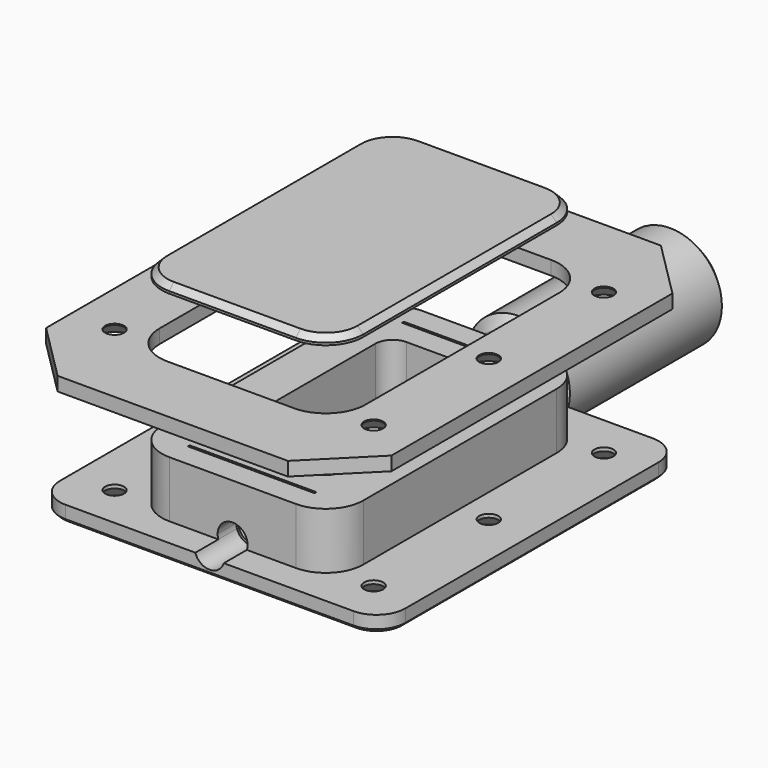
from build123d import *

# Parameters (mm, degrees)
F1_R          = 1.65
F2_DEPTH      = 2.8
F4_DEPTH      = 9.8
F6_DEPTH      = 65
F7_W          = 60
F7_H          = 81
F7_R          = 1.65
F8_DEPTH      = 2.4
F9_SIZE       = 10
F10_SIZE      = 2.2
F10_2_SIZE    = 2.2
F12_R         = 9
F12_R_2       = 2.7
F13_DEPTH     = 37
F14_SIZE      = 2
F16_SIZE      = 0.6
F19_DEPTH     = 1.4
F21_DEPTH     = 1.6
F22_W         = 11
F22_H         = 37.4000005722
F22_H_2       = 1.5999997139
F23_DEPTH     = 2
F24_SIZE      = 1.99999
F25_T1_DEPTH  = 38.2094607039
F25_T3_DEPTH  = 32
F25_T6_ANGLE  = 101.1642209188
F25_T8_ANGLE  = 101.1642209188
F25_T10_ANGLE = 101.1642209188
F25_T12_ANGLE = 101.1642209188
F26_SIZE      = 1
F27_W         = 22
F27_H         = 0.4
F28_DEPTH     = 12


# Not quite as in the source:
# - a fillet or chamfer that OpenCascade refuses, or shapes differently, is made with other operations: its cross-section is extruded or revolved along the edge and cut away or added
# - a fillet or chamfer is up to 0.001 mm smaller than in the source, because OpenCascade refuses the exact size


with BuildPart() as f2:
    # F1 (on Top) → F2 (new body)
    with BuildSketch(Plane.XY):
        with BuildLine():
            Line((25, 32.5), (-25, 32.5))
            ThreePointArc((-25, 32.5), (-28.5355339059, 31.0355339059), (-30, 27.5))
            Line((-30, 27.5), (-30, -27.5))
            ThreePointArc((-30, -27.5), (-28.5355339059, -31.0355339059), (-25, -32.5))
            Line((-25, -32.5), (25, -32.5))
            ThreePointArc((25, -32.5), (28.5355339059, -31.0355339059), (30, -27.5))
            Line((30, -27.5), (30, 27.5))
            ThreePointArc((30, 27.5), (28.5355339059, 31.0355339059), (25, 32.5))
        make_face()
        with Locations((-22.5, -25)):
            Circle(F1_R, mode=Mode.SUBTRACT)
        with Locations((22.5, -25)):
            Circle(F1_R, mode=Mode.SUBTRACT)
        with Locations((-22.5, 0)):
            Circle(F1_R, mode=Mode.SUBTRACT)
        with Locations((-22.5, 25)):
            Circle(F1_R, mode=Mode.SUBTRACT)
        with BuildLine():
            ThreePointArc((-10, 16), (-9.1213203436, 18.1213203436), (-7, 19))
            Line((-7, 19), (7, 19))
            ThreePointArc((7, 19), (9.1213203436, 18.1213203436), (10, 16))
            Line((10, 16), (10, -16))
            ThreePointArc((10, -16), (9.1213203436, -18.1213203436), (7, -19))
            Line((7, -19), (-7, -19))
            ThreePointArc((-7, -19), (-9.1213203436, -18.1213203436), (-10, -16))
            Line((-10, -16), (-10, 16))
        make_face(mode=Mode.SUBTRACT)
        with Locations((22.5, 0)):
            Circle(F1_R, mode=Mode.SUBTRACT)
        with Locations((22.5, 25)):
            Circle(F1_R, mode=Mode.SUBTRACT)
    extrude(amount=F2_DEPTH)

    # F3 (on face) → F4 (join)
    with BuildSketch(Plane.XY.offset(2.8)):
        with BuildLine():
            Line((11, 27.5), (-11, 27.5))
            ThreePointArc((-11, 27.5), (-15.5961940777, 25.5961940777), (-17.5, 21))
            Line((-17.5, 21), (-17.5, -21))
            ThreePointArc((-17.5, -21), (-15.5961940777, -25.5961940777), (-11, -27.5))
            Line((-11, -27.5), (11, -27.5))
            ThreePointArc((11, -27.5), (15.5961940777, -25.5961940777), (17.5, -21))
            Line((17.5, -21), (17.5, 21))
            ThreePointArc((17.5, 21), (15.5961940777, 25.5961940777), (11, 27.5))
        make_face()
        with BuildLine():
            Line((-10, -16), (-10, 16))
            ThreePointArc((-10, 16), (-9.1213203436, 18.1213203436), (-7, 19))
            Line((-7, 19), (7, 19))
            ThreePointArc((7, 19), (9.1213203436, 18.1213203436), (10, 16))
            Line((10, 16), (10, -16))
            ThreePointArc((10, -16), (9.1213203436, -18.1213203436), (7, -19))
            Line((7, -19), (-7, -19))
            ThreePointArc((-7, -19), (-9.1213203436, -18.1213203436), (-10, -16))
        make_face(mode=Mode.SUBTRACT)
    extrude(amount=F4_DEPTH)

    # F5 (on face) → F6 (cut, through all)
    with BuildSketch(Plane.XZ.offset(32.5)):
        with BuildLine():
            ThreePointArc((2.6, 3.6), (0, 6.2), (-2.6, 3.6))
            Line((-2.6, 3.6), (2.6, 3.6))
        make_face()
        with BuildLine():
            Line((2.6, 3.6), (-2.6, 3.6))
            ThreePointArc((-2.6, 3.6), (-2.5682722574, 3.1950585079), (-2.4738633754, 2.8))
            Line((-2.4738633754, 2.8), (2.4738633754, 2.8))
            ThreePointArc((2.4738633754, 2.8), (2.5682722574, 3.1950585079), (2.6, 3.6))
        make_face()
        with BuildLine():
            Line((2.4738633754, 2.8), (-2.4738633754, 2.8))
            ThreePointArc((-2.4738633754, 2.8), (0, 1), (2.4738633754, 2.8))
        make_face()
    extrude(amount=-F6_DEPTH, mode=Mode.SUBTRACT)

    # F10
    f10_edges = [f2.edges().sort_by_distance(p)[0] for p in [
        (-24.15, -25, 0),
        (-24.15, 25, 0),
        (20.85, 25, 0),
        (20.85, -25, 0),
        (20.85, 0, 0),
        (-24.15, 0, 0),
    ]]
    chamfer(f10_edges, length=F10_SIZE)

    # F16
    f16_edges = [f2.edges().sort_by_distance(p)[0] for p in [
        (0, -32.5, 0),
        (-10, 0, 0),
        (-28.535534, 31.035534, 0),
        (-30, 0, 0),
        (-28.535534, -31.035534, 0),
        (28.535534, -31.035534, 0),
        (30, 0, 0),
        (28.535534, 31.035534, 0),
        (-9.12132, 18.12132, 0),
        (0, 19, 0),
        (9.12132, 18.12132, 0),
        (10, 0, 0),
        (9.12132, -18.12132, 0),
        (0, -19, 0),
        (-9.12132, -18.12132, 0),
    ]]
    chamfer(f16_edges, length=F16_SIZE)

    # F27 (on face) → F28 (cut)
    with BuildSketch(Plane.XY.offset(12.6)):
        with Locations((0, 23.25)):
            Rectangle(F27_W, F27_H)
        with Locations((0, -23.25)):
            Rectangle(F27_W, F27_H)
    extrude(amount=-F28_DEPTH, mode=Mode.SUBTRACT)


with BuildPart() as f8:
    # F7 (on offset) → F8 (new body)
    with BuildSketch(Plane.XY.offset(25)):
        Rectangle(F7_W, F7_H)
        with Locations((-22.5, -25)):
            Circle(F7_R, mode=Mode.SUBTRACT)
        with Locations((22.5, -25)):
            Circle(F7_R, mode=Mode.SUBTRACT)
        with Locations((-22.5, 0)):
            Circle(F7_R, mode=Mode.SUBTRACT)
        with Locations((-22.5, 25)):
            Circle(F7_R, mode=Mode.SUBTRACT)
        with BuildLine():
            ThreePointArc((-17.9, 21), (-15.8790367902, 25.8790367902), (-11, 27.9))
            Line((-11, 27.9), (11, 27.9))
            ThreePointArc((11, 27.9), (15.8790367902, 25.8790367902), (17.9, 21))
            Line((17.9, 21), (17.9, -21))
            ThreePointArc((17.9, -21), (15.8790367902, -25.8790367902), (11, -27.9))
            Line((11, -27.9), (-11, -27.9))
            ThreePointArc((-11, -27.9), (-15.8790367902, -25.8790367902), (-17.9, -21))
            Line((-17.9, -21), (-17.9, 21))
        make_face(mode=Mode.SUBTRACT)
        with Locations((22.5, 0)):
            Circle(F7_R, mode=Mode.SUBTRACT)
        with Locations((22.5, 25)):
            Circle(F7_R, mode=Mode.SUBTRACT)
    extrude(amount=F8_DEPTH)

    # F9
    f9_edges = [f8.edges().sort_by_distance(p)[0] for p in [
        (30, -40.5, 26.2),
        (30, 40.5, 26.2),
        (-30, 40.5, 26.2),
        (-30, -40.5, 26.2),
    ]]
    chamfer(f9_edges, length=F9_SIZE)

    # F10#2
    f10_2_edges = [f8.edges().sort_by_distance(p)[0] for p in [
        (20.85, -25, 25),
        (20.85, 0, 25),
        (20.85, 25, 25),
        (-24.15, 25, 25),
        (-24.15, 0, 25),
        (-24.15, -25, 25),
    ]]
    chamfer(f10_2_edges, length=F10_2_SIZE)


with BuildPart() as f13:
    # F12 (on offset) → F13 (new body)
    with BuildSketch(Plane.XZ.offset(-69.5)):
        with Locations((0, 3.6)):
            Circle(F12_R)
        with Locations((0, 3.6)):
            Circle(F12_R_2, mode=Mode.SUBTRACT)
    extrude(amount=F13_DEPTH)

    # F14
    f14_edges = [f13.edges().sort_by_distance(p)[0] for p in [
        (-9, 69.5, 3.6),
        (-9, 32.5, 3.6),
    ]]
    chamfer(f14_edges, length=F14_SIZE)

    # F15: chamfer of 0.4 on 4 edges, made by hand

    # F15_s1 → F15_t2 (revolve, cut)
    with BuildSketch(Plane.XY.offset(3.6)):
        Polygon((7.1171572875, 69.3828427125), (6.8343145751, 69.5), (7, 69.5), align=None)
    revolve(axis=Axis((0, 69.5, 3.6), (0, -1, 0)), mode=Mode.SUBTRACT)

    # F15_s3 → F15_t4 (revolve, cut)
    with BuildSketch(Plane.XY.offset(3.6)):
        Polygon((3.1, 69.5), (2.7, 69.1), (2.7, 69.5), align=None)
    revolve(axis=Axis((0, 69.5, 3.6), (0, -1, 0)), mode=Mode.SUBTRACT)

    # F15_s5 → F15_t6 (revolve, cut)
    with BuildSketch(Plane.XY.offset(3.6)):
        Polygon((7.1171572875, 32.6171572875), (6.8343145751, 32.5), (7, 32.5), align=None)
    revolve(axis=Axis((0, 32.5, 3.6), (0, -1, 0)), mode=Mode.SUBTRACT)

    # F15_s7 → F15_t8 (revolve, cut)
    with BuildSketch(Plane.XY.offset(3.6)):
        Polygon((3.1, 32.5), (2.7, 32.9), (2.7, 32.5), align=None)
    revolve(axis=Axis((0, 32.5, 3.6), (0, -1, 0)), mode=Mode.SUBTRACT)


with BuildPart() as f19:
    # F18 (on offset) → F19 (new body)
    with BuildSketch(Plane.XY.offset(37.6)):
        with BuildLine():
            Line((-17.5, 21), (-17.5, -21))
            ThreePointArc((-17.5, -21), (-15.5961940777, -25.5961940777), (-11, -27.5))
            Line((-11, -27.5), (11, -27.5))
            ThreePointArc((11, -27.5), (15.5961940777, -25.5961940777), (17.5, -21))
            Line((17.5, -21), (17.5, 21))
            ThreePointArc((17.5, 21), (15.5961940777, 25.5961940777), (11, 27.5))
            Line((11, 27.5), (-11, 27.5))
            ThreePointArc((-11, 27.5), (-15.5961940777, 25.5961940777), (-17.5, 21))
        make_face()
    extrude(amount=F19_DEPTH)

    # F20 (on face) → F21 (join)
    with BuildSketch(Plane(origin=(0, 0, 37.6), x_dir=(1, 0, 0), z_dir=(0, 0, -1))):
        with BuildLine():
            ThreePointArc((-9.7000002861, -16), (-8.9091885115, -17.9091885115), (-7, -18.7000002861))
            Line((-7, -18.7000002861), (7, -18.7000002861))
            ThreePointArc((7, -18.7000002861), (8.9091885115, -17.9091885115), (9.7000002861, -16))
            Line((9.7000002861, -16), (9.7000002861, 16))
            ThreePointArc((9.7000002861, 16), (8.9091885115, 17.9091885115), (7, 18.7000002861))
            Line((7, 18.7000002861), (-7, 18.7000002861))
            ThreePointArc((-7, 18.7000002861), (-8.9091885115, 17.9091885115), (-9.7000002861, 16))
            Line((-9.7000002861, 16), (-9.7000002861, -16))
        make_face()
    extrude(amount=F21_DEPTH)

    # F22 (on face) → F23 (cut)
    with BuildSketch(Plane(origin=(0, 0, 36), x_dir=(1, 0, 0), z_dir=(0, 0, -1))):
        Rectangle(F22_W, F22_H)
        with Locations((0, 19.5000001431)):
            Rectangle(F22_W, F22_H_2)
        with Locations((0, -19.5000001431)):
            Rectangle(F22_W, F22_H_2)
    extrude(amount=-F23_DEPTH, mode=Mode.SUBTRACT)

    # F24 (call 1 of 2: OpenCascade refuses the feature's edges together) (size 2 in the source; OpenCascade refuses exactly that, so slightly less here)
    f24_edges = [f19.edges().sort_by_distance(p)[0] for p in [
        (-5.5, 0, 36),
    ]]
    chamfer(f24_edges, length=F24_SIZE)

    # F24#2 (call 2 of 2) (size 2 in the source; OpenCascade refuses exactly that, so slightly less here)
    f24_2_edges = [f19.edges().sort_by_distance(p)[0] for p in [
        (5.5, 0, 36),
    ]]
    chamfer(f24_2_edges, length=F24_SIZE)

    # F25: chamfer of 0.4 on 8 edges, made by hand

    # F25_s2 → F25_t1 (cut)
    with BuildSketch(Plane.XZ.offset(-19.1047303519)):
        Polygon((-7.3828327125, 36.1171572875), (-7.6656754249, 36), (-7.49999, 36), align=None)
        Polygon((7.3828327125, 36.1171572875), (7.6656754249, 36), (7.49999, 36), align=None)
    extrude(amount=F25_T1_DEPTH, mode=Mode.SUBTRACT)

    # F25_s4 → F25_t3 (cut)
    with BuildSketch(Plane.XZ.offset(-16)):
        Polygon((-9.7000002861, 36.4), (-9.3000002861, 36), (-9.7000002861, 36), align=None)
        Polygon((9.7000002861, 36.4), (9.3000002861, 36), (9.7000002861, 36), align=None)
    extrude(amount=F25_T3_DEPTH, mode=Mode.SUBTRACT)

    # F25_s5 → F25_t6 (revolve, cut)
    with BuildSketch(Plane(origin=(-9.7768974657, -1.9295339384, 0), x_dir=(0, 0, 1), z_dir=(0.9810762562, 0.1936217434, 0))):
        Polygon((36.4, 17.0418681814), (36, 16.6418681814), (36, 17.0418681814), align=None)
    revolve(axis=Axis((-7, -16, 36), (0, 0, -1)), revolution_arc=F25_T6_ANGLE, mode=Mode.SUBTRACT)

    # F25_s7 → F25_t8 (revolve, cut)
    with BuildSketch(Plane.XZ.offset(-16)):
        Polygon((-9.7000002861, 36.4), (-9.3000002861, 36), (-9.7000002861, 36), align=None)
    revolve(axis=Axis((-7, 16, 36), (0, 0, -1)), revolution_arc=F25_T8_ANGLE, mode=Mode.SUBTRACT)

    # F25_s9 → F25_t10 (revolve, cut)
    with BuildSketch(Plane.XZ.offset(16)):
        Polygon((9.7000002861, 36.4), (9.3000002861, 36), (9.7000002861, 36), align=None)
    revolve(axis=Axis((7, -16, 36), (0, 0, -1)), revolution_arc=F25_T10_ANGLE, mode=Mode.SUBTRACT)

    # F25_s11 → F25_t12 (revolve, cut)
    with BuildSketch(Plane(origin=(9.7768974657, 1.9295339384, 0), x_dir=(0, 0, 1), z_dir=(-0.9810762562, -0.1936217434, 0))):
        Polygon((36.4, 17.0418681814), (36, 16.6418681814), (36, 17.0418681814), align=None)
    revolve(axis=Axis((7, 16, 36), (0, 0, -1)), revolution_arc=F25_T12_ANGLE, mode=Mode.SUBTRACT)

    # F26
    f26_edges = [f19.edges().sort_by_distance(p)[0] for p in [
        (-17.5, 0, 39),
        (-15.596194, -25.596194, 39),
        (0, -27.5, 39),
        (15.596194, -25.596194, 39),
        (17.5, 0, 39),
        (15.596194, 25.596194, 39),
        (0, 27.5, 39),
        (-15.596194, 25.596194, 39),
    ]]
    chamfer(f26_edges, length=F26_SIZE)


solid = Compound([f2.part, f8.part, f13.part, f19.part])
